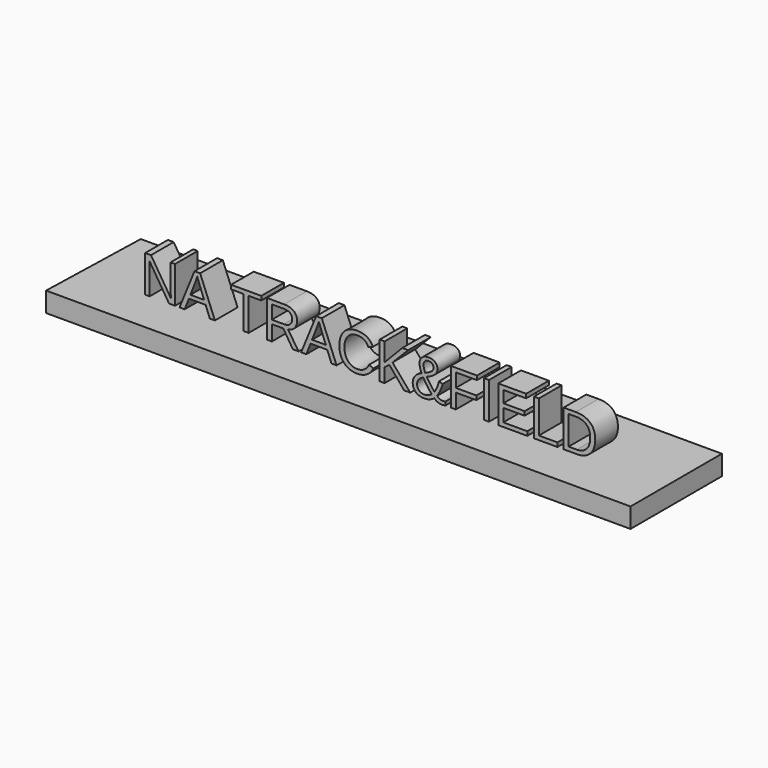
from build123d import *

# Parameters (mm, degrees)
F1_DEPTH     = 3.556
F2_TEXT_SIZE = 9.5797405164
F3_DEPTH     = 5.08


# Not quite as in the source:
# - Text() gives the source's letters only with a copy of the font that has no kerning and outlines rounded to 1/6400 em; it was checked with that copy


with BuildPart() as f1:
    # F0 (on Top) → F1 (new body)
    with BuildSketch(Plane.XY):
        Polygon((-52.3218102753, 7.9812929034), (-52.913017571, -12.5138796866), (51.9276745617, -12.5138796866), (51.9276745617, 7.9812929034), align=None)
    extrude(amount=F1_DEPTH)


with BuildPart() as f3:
    # F2 (on Front) → F3 (new body)
    with BuildSketch(Plane.XZ):
        with Locations((-41.8622046709, 3.7249065936)):
            Text('NA TRACK&FIELD', F2_TEXT_SIZE, font='Arimo', text_align=(TextAlign.LEFT, TextAlign.BOTTOM))
    extrude(amount=F3_DEPTH)


solid = Compound([f1.part, f3.part])
